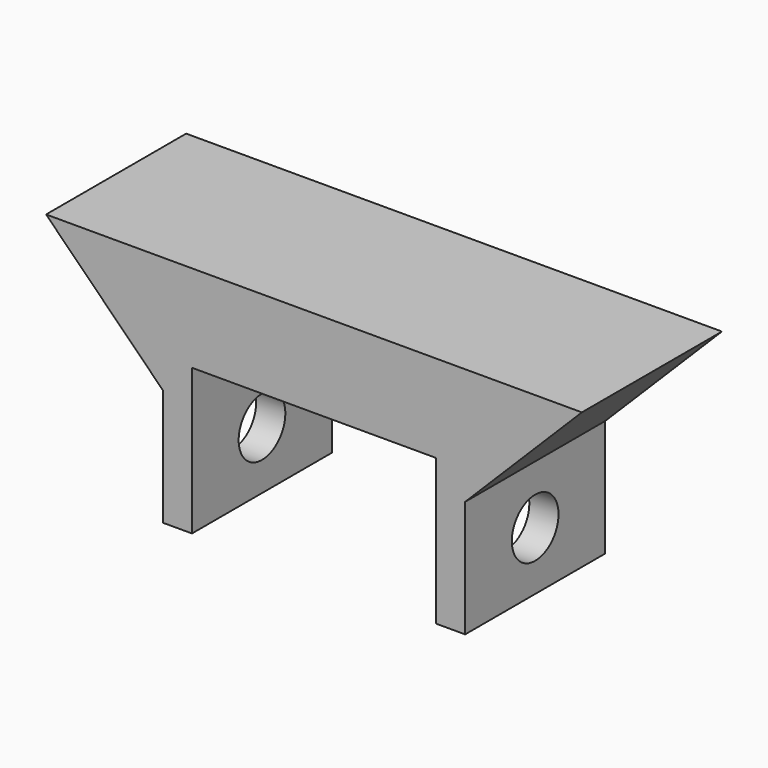
from build123d import *

# Parameters (mm, degrees)
F0_W        = 283.9974
F0_H        = 76.2
F1_DEPTH    = 50.8
F2_T1_DEPTH = 468.124487366
F3_DEPTH    = 50.8
F4_W        = 106.1974
F4_H        = 76.2
F5_DEPTH    = 63.5
F6_R        = 12.7
F7_DEPTH    = 182.3984


# Not quite as in the source:
# - a fillet or chamfer that OpenCascade refuses, or shapes differently, is made with other operations: its cross-section is extruded or revolved along the edge and cut away or added


with BuildPart() as f1:
    # F0 (on Top) → F1 (new body)
    with BuildSketch(Plane.XY):
        with Locations((141.9987, 38.1)):
            Rectangle(F0_W, F0_H)
    extrude(amount=-F1_DEPTH)

    # F2: chamfer of 76.2 on 2 edges, made by hand

    # F2_s2 → F2_t1 (cut)
    with BuildSketch(Plane.XZ.offset(-272.162243683)):
        Polygon((0, 25.4), (76.2, -50.8), (0, -50.8), align=None)
        Polygon((283.9974, 25.4), (207.7974, -50.8), (283.9974, -50.8), align=None)
    extrude(amount=F2_T1_DEPTH, mode=Mode.SUBTRACT)

    # F3 (add): a face of the model
    f3_faces = [f1.faces().sort_by_distance(p)[0] for p in [
        (141.9987, 38.1, -50.8),
    ]]
    extrude(f3_faces, amount=F3_DEPTH)

    # F4 (on face) → F5 (cut)
    with BuildSketch(Plane(origin=(0, 0, -101.6), x_dir=(1, 0, 0), z_dir=(0, 0, -1))):
        with Locations((141.9987, -38.1)):
            Rectangle(F4_W, F4_H)
    extrude(amount=-F5_DEPTH, mode=Mode.SUBTRACT)

    # F6 (on face) → F7 (cut, through all)
    with BuildSketch(Plane.YZ.offset(207.7974)):
        with Locations((38.1, -76.2)):
            Circle(F6_R)
    extrude(amount=-F7_DEPTH, mode=Mode.SUBTRACT)


solid = f1.part
